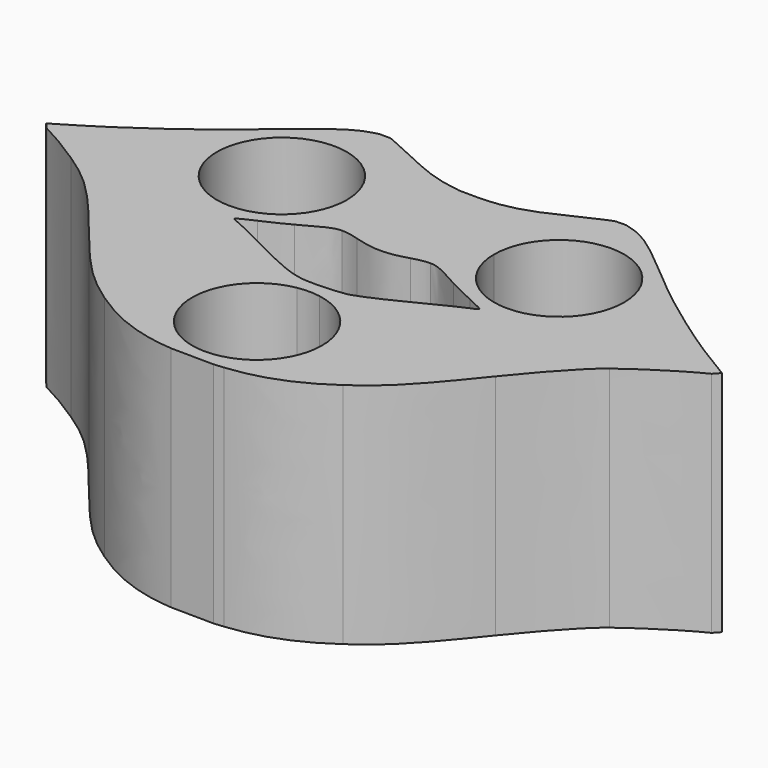
from build123d import *

# Parameters (mm, degrees)
F1_DEPTH = 25.4
F2_R     = 7.239
F3_DEPTH = 24.13


# Not quite as in the source:
# - ends of sketch curves that miss each other by under 0.0002 mm in the source are joined


with BuildPart() as f1:
    # F0 (on Top) → F1 (new body)
    with BuildSketch(Plane.XY):
        with BuildLine():
            add(Edge.make_bspline(
                [(-13.1884615385, -19.7055979293), (-9.7172457191, -22.0951789594), (-6.5189125485, -23.2662965046), (-2.6759197324, -23.5549250296)],
                knots=[0, 0, 0, 0, 1, 1, 1, 1], degree=3))
            Line((-2.6759197324, -23.5549250296), (2.1025083612, -23.6077884611))
            Line((2.1025083612, -23.6077884611), (3.1856187291, -23.5036646015))
            add(Edge.make_bspline(
                [(3.1856187291, -23.5036646015), (6.8168163211, -23.15457813), (9.9794896756, -21.9435460564), (13.3158862876, -19.6246398892)],
                knots=[0, 0, 0, 0, 1, 1, 1, 1], degree=3))
            add(Edge.make_bspline(
                [(13.3158862876, -19.6246398892), (16.4115571605, -17.4730475146), (17.9082372943, -15.9389605714), (22.6381101873, -10.0694262069)],
                knots=[0, 0, 0, 0, 1, 1, 1, 1], degree=3))
            add(Edge.make_bspline(
                [(22.6381101873, -10.0694262069), (25.5016513946, -6.5159182102), (27.9048694214, -3.927799227), (29.4743562341, -2.7072102972)],
                knots=[0, 0, 0, 0, 1, 1, 1, 1], degree=3))
            add(Edge.make_bspline(
                [(29.4743562341, -2.7072102972), (31.4678692876, -1.1568550363), (35.1474296689, 1.1661975322), (37.0124718161, 2.0519014787)],
                knots=[0, 0, 0, 0, 1, 1, 1, 1], degree=3))
            Line((37.0124718161, 2.0519014787), (37.6322441338, 2.7317278065))
            add(Edge.make_bspline(
                [(37.6322441338, 2.7317278065), (33.9167308595, 4.9403402078), (32.5687337458, 5.8151659035), (29.1802675585, 8.2169048474)],
                knots=[0, 0, 0, 0, 1, 1, 1, 1], degree=3))
            add(Edge.make_bspline(
                [(29.1802675585, 8.2169048474), (26.5643967391, 10.0710303571), (24.4979457592, 11.6894900051), (21.789632107, 14.0053073964)],
                knots=[0, 0, 0, 0, 1, 1, 1, 1], degree=3))
            add(Edge.make_bspline(
                [(21.789632107, 14.0053073964), (17.557108204, 17.6244421652), (16.0735171405, 18.6431407559), (14.3652864381, 19.1031879026)],
                knots=[0, 0, 0, 0, 1, 1, 1, 1], degree=3))
            Line((14.3652864381, 19.1031879026), (13.6981605351, 19.2828529762))
            Line((13.6981605351, 19.2828529762), (13.6904819746, 19.2842043089))
            Line((13.6904819746, 19.2842043089), (12.5617656785, 19.2709062892))
            Line((12.5617656785, 19.2709062892), (11.8505016722, 19.0057804423))
            add(Edge.make_bspline(
                [(11.8505016722, 19.0057804423), (11.394958194, 18.8359751773), (10.018770903, 18.2002029302), (8.7923076923, 17.5929531204)],
                knots=[0, 0, 0, 0, 1, 1, 1, 1], degree=3))
            add(Edge.make_bspline(
                [(8.7923076923, 17.5929531204), (5.3799595585, 15.9034224779), (3.4433187191, 15.3647120515), (0.5096989967, 15.2890007254)],
                knots=[0, 0, 0, 0, 1, 1, 1, 1], degree=3))
            add(Edge.make_bspline(
                [(0.5096989967, 15.2890007254), (-0.4364297659, 15.2645829578), (-1.411229097, 15.2701955402), (-1.6565217391, 15.3014730598)],
                knots=[0, 0, 0, 0, 1, 1, 1, 1], degree=3))
            add(Edge.make_bspline(
                [(-1.6565217391, 15.3014730598), (-4.1988442676, 15.625649745), (-5.7211355017, 16.1272113972), (-9.1745819398, 17.7785107923)],
                knots=[0, 0, 0, 0, 1, 1, 1, 1], degree=3))
            add(Edge.make_bspline(
                [(-9.1745819398, 17.7785107923), (-10.6112959866, 18.4654896305), (-11.9874832776, 19.0880385335), (-12.2327759197, 19.1619526928)],
                knots=[0, 0, 0, 0, 1, 1, 1, 1], degree=3))
            add(Edge.make_bspline(
                [(-12.2327759197, 19.1619526928), (-12.4038425542, 19.2135003349), (-12.5045889513, 19.2450051824), (-12.5224971626, 19.2615668616)],
                knots=[0, 0, 0, 0, 0.4016092701, 0.4016092701, 0.4016092701, 0.4016092701], degree=3))
            Line((-12.5224971626, 19.2615668616), (-13.7034814285, 19.2814199953))
            Line((-13.7034814285, 19.2814199953), (-14.3652864381, 19.1031879026))
            add(Edge.make_bspline(
                [(-14.3652864381, 19.1031879026), (-15.9654584047, 18.6722420201), (-17.5656112575, 17.5873902337), (-21.4073578595, 14.3288910786)],
                knots=[0, 0, 0, 0, 1, 1, 1, 1], degree=3))
            add(Edge.make_bspline(
                [(-21.4073578595, 14.3288910786), (-24.8686676789, 11.3930710494), (-26.1926326442, 10.347677133), (-28.8684434285, 8.4376666326)],
                knots=[0, 0, 0, 0, 1, 1, 1, 1], degree=3))
            add(Edge.make_bspline(
                [(-28.8684434285, 8.4376666326), (-32.2200301856, 6.0452835322), (-33.9212185999, 4.9376719336), (-37.6322438152, 2.7317278065)],
                knots=[0, 0, 0, 0, 1, 1, 1, 1], degree=3))
            Line((-37.6322438152, 2.7317278065), (-37.0124719753, 2.0519014787))
            add(Edge.make_bspline(
                [(-37.0124719753, 2.0519014787), (-35.8599579657, 1.5045752279), (-33.7339199875, 0.2440615757), (-31.856187291, -1.0052246818)],
                knots=[0, 0, 0, 0, 1, 1, 1, 1], degree=3))
            add(Edge.make_bspline(
                [(-31.856187291, -1.0052246818), (-28.3890610096, -3.3119617855), (-26.7945040146, -4.8987439594), (-22.168989602, -10.6451911133)],
                knots=[0, 0, 0, 0, 1, 1, 1, 1], degree=3))
            add(Edge.make_bspline(
                [(-22.168989602, -10.6451911133), (-17.8793743144, -15.9743400531), (-16.3129253077, -17.5547216818), (-13.1884615385, -19.7055979293)],
                knots=[0, 0, 0, 0, 1, 1, 1, 1], degree=3))
        make_face()
        with BuildLine():
            add(Edge.make_bspline(
                [(3.1856187291, -5.9524701801), (2.2569598997, -6.2331244644), (-0.9628468896, -6.3803357286), (-2.1025083612, -6.1942458992)],
                knots=[0, 0, 0, 0, 1, 1, 1, 1], degree=3))
            add(Edge.make_bspline(
                [(-2.1025083612, -6.1942458992), (-3.6078737659, -5.9484422838), (-5.1525675452, -5.2953738791), (-9.4931438127, -3.0696215748)],
                knots=[0, 0, 0, 0, 1, 1, 1, 1], degree=3))
            add(Edge.make_bspline(
                [(-9.4931438127, -3.0696215748), (-11.0349832776, -2.2789994276), (-12.5975292642, -1.5271169527), (-12.9654682274, -1.3987709226)],
                knots=[0, 0, 0, 0, 1, 1, 1, 1], degree=3))
            add(Edge.make_bspline(
                [(-12.9654682274, -1.3987709226), (-13.3334071906, -1.2704261668), (-13.6344481605, -1.1015348557), (-13.6344481605, -1.0234578892)],
                knots=[0, 0, 0, 0, 1, 1, 1, 1], degree=3))
            add(Edge.make_bspline(
                [(-13.6344481605, -1.0234578892), (-13.6344481605, -0.9453809226), (-12.8145884047, -0.5248066183), (-11.8125380167, -0.0888470497)],
                knots=[0, 0, 0, 0, 1, 1, 1, 1], degree=3))
            add(Edge.make_bspline(
                [(-11.8125380167, -0.0888470497), (-10.810488903, 0.3471112446), (-9.4773074649, 0.9934414286), (-8.8499125987, 1.3474413985)],
                knots=[0, 0, 0, 0, 1, 1, 1, 1], degree=3))
            add(Edge.make_bspline(
                [(-8.8499125987, 1.3474413985), (-6.2956095953, 2.7886790239), (-5.7246919264, 3.0341564319), (-4.9058528428, 3.04326985)],
                knots=[0, 0, 0, 0, 1, 1, 1, 1], degree=3))
            add(Edge.make_bspline(
                [(-4.9058528428, 3.04326985), (-4.4052494247, 3.0488383115), (-3.7453867324, 2.9284155523), (-2.9944816054, 2.6944458734)],
                knots=[0, 0, 0, 0, 1, 1, 1, 1], degree=3))
            add(Edge.make_bspline(
                [(-2.9944816054, 2.6944458734), (-0.8245757458, 2.0183365255), (0.8245757458, 2.0183365255), (2.9944816054, 2.6944458734)],
                knots=[0, 0, 0, 0, 1, 1, 1, 1], degree=3))
            add(Edge.make_bspline(
                [(2.9944816054, 2.6944458734), (3.7453867324, 2.9284155523), (4.4052494247, 3.04884086), (4.9058528428, 3.04326985)],
                knots=[0, 0, 0, 0, 1, 1, 1, 1], degree=3))
            add(Edge.make_bspline(
                [(4.9058528428, 3.04326985), (5.7246919264, 3.0341589804), (6.2956095953, 2.7886790239), (8.8499125987, 1.3474413985)],
                knots=[0, 0, 0, 0, 1, 1, 1, 1], degree=3))
            add(Edge.make_bspline(
                [(8.8499125987, 1.3474413985), (9.4773074649, 0.9934414286), (10.810488903, 0.3471112446), (11.8125380167, -0.0888470497)],
                knots=[0, 0, 0, 0, 1, 1, 1, 1], degree=3))
            add(Edge.make_bspline(
                [(11.8125380167, -0.0888470497), (12.8145884047, -0.5248066183), (13.6344481605, -0.9453809226), (13.6344481605, -1.0234578892)],
                knots=[0, 0, 0, 0, 1, 1, 1, 1], degree=3))
            add(Edge.make_bspline(
                [(13.6344481605, -1.0234578892), (13.6344481605, -1.1015348557), (13.3334071906, -1.2702719828), (12.9654682274, -1.39842815)],
                knots=[0, 0, 0, 0, 1, 1, 1, 1], degree=3))
            add(Edge.make_bspline(
                [(12.9654682274, -1.39842815), (12.5975292642, -1.5265855915), (11.0903047324, -2.2520210597), (9.616079388, -3.0105054109)],
                knots=[0, 0, 0, 0, 1, 1, 1, 1], degree=3))
            add(Edge.make_bspline(
                [(9.616079388, -3.0105054109), (6.4728204682, -4.6277051467), (4.3392408562, -5.6038271467), (3.1856187291, -5.9524701801)],
                knots=[0, 0, 0, 0, 1, 1, 1, 1], degree=3))
        make_face(mode=Mode.SUBTRACT)
    extrude(amount=F1_DEPTH)

    # F2 (on face) → F3 (cut)
    with BuildSketch(Plane.XY.offset(25.4)):
        with BuildLine():
            Line((-15.4391787946, 0.5730026737), (-15.4391787946, 7.8120026737))
            Line((-15.4391787946, 7.8120026737), (-8.2001787946, 7.8120026737))
            ThreePointArc((-8.2001787946, 7.8120026737), (-20.5579247836, 12.9307486628), (-15.4391787946, 0.5730026737))
        make_face()
        with BuildLine():
            Line((-8.2001787946, 7.8120026737), (-15.4391787946, 7.8120026737))
            Line((-15.4391787946, 7.8120026737), (-15.4391787946, 0.5730026737))
            ThreePointArc((-15.4391787946, 0.5730026737), (-10.3204328056, 2.6932566847), (-8.2001787946, 7.8120026737))
        make_face()
        with BuildLine():
            ThreePointArc((5.2293543768, 16.0678049121), (0.0138821984, 18.3010974633), (-5.2101171545, 16.0878246774))
            add(Edge.make_bspline(
                [(-1.6565217391, 15.3014730598), (-2.9785522156, 15.4700478385), (-4.0247567323, 15.686589164), (-5.2101171545, 16.0878246774)],
                knots=[0, 0, 0, 0, 0.5200089531, 0.5200089531, 0.5200089531, 0.5200089531], degree=3))
            add(Edge.make_bspline(
                [(0.5096989967, 15.2890007254), (-0.4364297659, 15.2645829578), (-1.411229097, 15.2701955402), (-1.6565217391, 15.3014730598)],
                knots=[0, 0, 0, 0, 1, 1, 1, 1], degree=3))
            add(Edge.make_bspline(
                [(5.2293543768, 16.0678049121), (3.6603216323, 15.5449011909), (2.2630856254, 15.3342524074), (0.5096989967, 15.2890007254)],
                knots=[0.4023129122, 0.4023129122, 0.4023129122, 0.4023129122, 1, 1, 1, 1], degree=3))
        make_face()
        with BuildLine():
            add(Edge.make_bspline(
                [(-13.4162854763, -0.8613894905), (-13.1075898138, -0.6826431402), (-12.5033600683, -0.3894012805), (-11.8125380167, -0.0888470497)],
                knots=[0.3105915033, 0.3105915033, 0.3105915033, 0.3105915033, 1, 1, 1, 1], degree=3))
            ThreePointArc((-13.4162854763, -0.8613894905), (-11.8071303692, -1.5501063766), (-10.4103203839, -2.6049205653))
            add(Edge.make_bspline(
                [(-9.4931438127, -3.0696215748), (-9.8012757449, -2.911618141), (-10.1102346708, -2.7551619236), (-10.4103203839, -2.6049205653)],
                knots=[0, 0, 0, 0, 0.1998469615, 0.1998469615, 0.1998469615, 0.1998469615], degree=3))
            add(Edge.make_bspline(
                [(-2.1025083612, -6.1942458992), (-3.6078737659, -5.9484422838), (-5.1525675452, -5.2953738791), (-9.4931438127, -3.0696215748)],
                knots=[0, 0, 0, 0, 1, 1, 1, 1], degree=3))
            add(Edge.make_bspline(
                [(3.1856187291, -5.9524701801), (2.2569598997, -6.2331244644), (-0.9628468896, -6.3803357286), (-2.1025083612, -6.1942458992)],
                knots=[0, 0, 0, 0, 1, 1, 1, 1], degree=3))
            add(Edge.make_bspline(
                [(9.616079388, -3.0105054109), (6.4728204682, -4.6277051467), (4.3392408562, -5.6038271467), (3.1856187291, -5.9524701801)],
                knots=[0, 0, 0, 0, 1, 1, 1, 1], degree=3))
            add(Edge.make_bspline(
                [(10.4068537547, -2.6082707732), (10.1467262743, -2.7391031612), (9.8808705361, -2.8742711894), (9.616079388, -3.0105054109)],
                knots=[0.8203862462, 0.8203862462, 0.8203862462, 0.8203862462, 1, 1, 1, 1], degree=3))
            ThreePointArc((10.4068537547, -2.6082707732), (11.8050454626, -1.5513161359), (13.4162854763, -0.8613894905))
            add(Edge.make_bspline(
                [(11.8125380167, -0.0888470497), (12.5033600683, -0.3894012805), (13.1075898138, -0.6826431402), (13.4162854763, -0.8613894905)],
                knots=[0, 0, 0, 0, 0.6894084967, 0.6894084967, 0.6894084967, 0.6894084967], degree=3))
            add(Edge.make_bspline(
                [(8.8499125987, 1.3474413985), (9.4773074649, 0.9934414286), (10.810488903, 0.3471112446), (11.8125380167, -0.0888470497)],
                knots=[0, 0, 0, 0, 1, 1, 1, 1], degree=3))
            add(Edge.make_bspline(
                [(4.9058528428, 3.04326985), (5.7246919264, 3.0341589804), (6.2956095953, 2.7886790239), (8.8499125987, 1.3474413985)],
                knots=[0, 0, 0, 0, 1, 1, 1, 1], degree=3))
            add(Edge.make_bspline(
                [(2.9944816054, 2.6944458734), (3.7453867324, 2.9284155523), (4.4052494247, 3.04884086), (4.9058528428, 3.04326985)],
                knots=[0, 0, 0, 0, 1, 1, 1, 1], degree=3))
            add(Edge.make_bspline(
                [(-2.9944816054, 2.6944458734), (-0.8245757458, 2.0183365255), (0.8245757458, 2.0183365255), (2.9944816054, 2.6944458734)],
                knots=[0, 0, 0, 0, 1, 1, 1, 1], degree=3))
            add(Edge.make_bspline(
                [(-4.9058528428, 3.04326985), (-4.4052494247, 3.0488383115), (-3.7453867324, 2.9284155523), (-2.9944816054, 2.6944458734)],
                knots=[0, 0, 0, 0, 1, 1, 1, 1], degree=3))
            add(Edge.make_bspline(
                [(-8.8499125987, 1.3474413985), (-6.2956095953, 2.7886790239), (-5.7246919264, 3.0341564319), (-4.9058528428, 3.04326985)],
                knots=[0, 0, 0, 0, 1, 1, 1, 1], degree=3))
            add(Edge.make_bspline(
                [(-11.8125380167, -0.0888470497), (-10.810488903, 0.3471112446), (-9.4773074649, 0.9934414286), (-8.8499125987, 1.3474413985)],
                knots=[0, 0, 0, 0, 1, 1, 1, 1], degree=3))
        make_face()
        with BuildLine():
            ThreePointArc((-10.4103203839, -2.6049205653), (-11.8071303692, -1.5501063766), (-13.4162854763, -0.8613894905))
            add(Edge.make_bspline(
                [(-13.6344481605, -1.0234578892), (-13.6344481605, -0.9992078468), (-13.5553586823, -0.9419180856), (-13.4162854763, -0.8613894905)],
                knots=[0, 0, 0, 0, 0.3105915033, 0.3105915033, 0.3105915033, 0.3105915033], degree=3))
            add(Edge.make_bspline(
                [(-12.9654682274, -1.3987709226), (-13.3334071906, -1.2704261668), (-13.6344481605, -1.1015348557), (-13.6344481605, -1.0234578892)],
                knots=[0, 0, 0, 0, 1, 1, 1, 1], degree=3))
            add(Edge.make_bspline(
                [(-10.4103203839, -2.6049205653), (-11.6118122322, -2.003379874), (-12.671060748, -1.5014673886), (-12.9654682274, -1.3987709226)],
                knots=[0.1998469615, 0.1998469615, 0.1998469615, 0.1998469615, 1, 1, 1, 1], degree=3))
        make_face()
        with BuildLine():
            ThreePointArc((22.6781787946, 7.8120026737), (15.4391787946, 15.0510026737), (8.2001787946, 7.8120026737))
            Line((8.2001787946, 7.8120026737), (15.4391787946, 7.8120026737))
            Line((15.4391787946, 7.8120026737), (15.4391787946, 0.5730026737))
            ThreePointArc((15.4391787946, 0.5730026737), (20.5579247836, 2.6932566847), (22.6781787946, 7.8120026737))
        make_face()
        with BuildLine():
            Line((15.4391787946, 7.8120026737), (8.2001787946, 7.8120026737))
            ThreePointArc((8.2001787946, 7.8120026737), (10.3204328056, 2.6932566847), (15.4391787946, 0.5730026737))
            Line((15.4391787946, 0.5730026737), (15.4391787946, 7.8120026737))
        make_face()
        with BuildLine():
            ThreePointArc((1.2698828628, -7.8120026737), (0, -7.699749373), (-1.2698828628, -7.8120026737))
            Line((-1.2698828628, -7.8120026737), (1.2698828628, -7.8120026737))
        make_face()
        with BuildLine():
            Line((1.2698828628, -7.8120026737), (-1.2698828628, -7.8120026737))
            ThreePointArc((-1.2698828628, -7.8120026737), (-4.648141508, -20.4883350802), (7.239, -14.938749373))
            ThreePointArc((7.239, -14.938749373), (5.5495857072, -10.290607865), (1.2698828628, -7.8120026737))
        make_face()
        with BuildLine():
            add(Edge.make_bspline(
                [(13.4162854763, -0.8613894905), (13.5553586823, -0.9419180856), (13.6344481605, -0.9992078468), (13.6344481605, -1.0234578892)],
                knots=[0.6894084967, 0.6894084967, 0.6894084967, 0.6894084967, 1, 1, 1, 1], degree=3))
            ThreePointArc((13.4162854763, -0.8613894905), (11.8050454626, -1.5513161359), (10.4068537547, -2.6082707732))
            add(Edge.make_bspline(
                [(12.9654682274, -1.39842815), (12.6636161626, -1.5035667524), (11.5949866381, -2.010693531), (10.4068537547, -2.6082707732)],
                knots=[0, 0, 0, 0, 0.8203862462, 0.8203862462, 0.8203862462, 0.8203862462], degree=3))
            add(Edge.make_bspline(
                [(13.6344481605, -1.0234578892), (13.6344481605, -1.1015348557), (13.3334071906, -1.2702719828), (12.9654682274, -1.39842815)],
                knots=[0, 0, 0, 0, 1, 1, 1, 1], degree=3))
        make_face()
        with Locations((-53.0695078206, 0)):
            Circle(F2_R)
        with Locations((49.2036237652, 0)):
            Circle(F2_R)
    extrude(amount=-F3_DEPTH, mode=Mode.SUBTRACT)


solid = f1.part
